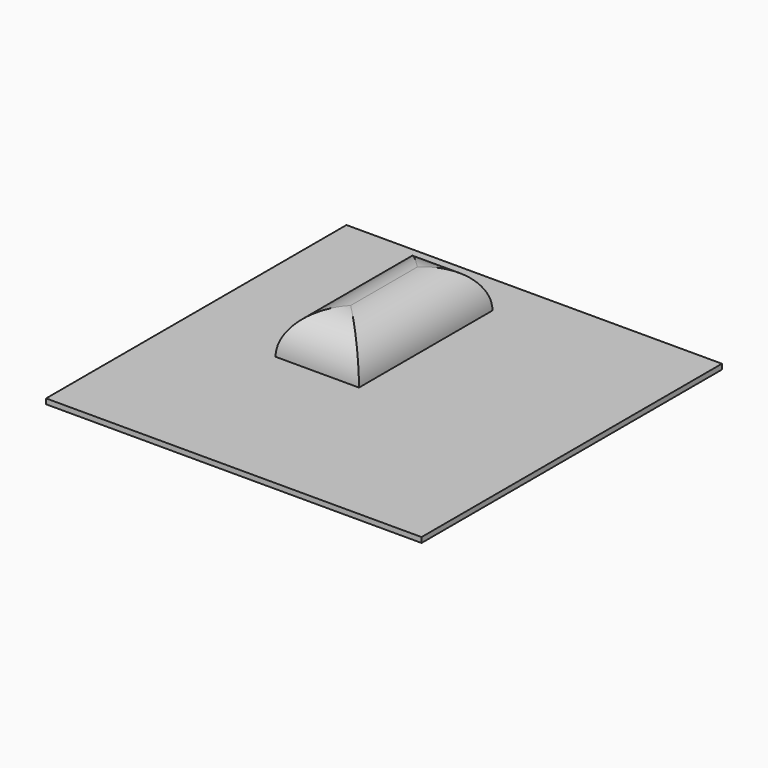
from build123d import *

# Parameters (mm, degrees)
F0_W     = 50.8
F0_H     = 101.6
F1_DEPTH = 25.4
F2_R     = 25.39999
F4_W     = 228.6
F4_H     = 228.6
F5_DEPTH = 3.175


# Not quite as in the source:
# - a fillet or chamfer is up to 0.001 mm smaller than in the source, because OpenCascade refuses the exact size


with BuildPart() as f1:
    # F0 (on Top) → F1 (new body)
    with BuildSketch(Plane.XY):
        Rectangle(F0_W, F0_H)
    extrude(amount=F1_DEPTH)

    # F2 (radius 25.4 in the source; OpenCascade refuses exactly that, so slightly less here)
    f2_edges = [f1.edges().sort_by_distance(p)[0] for p in [
        (-25.4, 0, 25.4),
        (0, -50.8, 25.4),
        (25.4, 0, 25.4),
        (0, 50.8, 25.4),
    ]]
    fillet(f2_edges, radius=F2_R)


with BuildPart() as f5:
    # F4 (on offset) → F5 (new body)
    with BuildSketch(Plane.XY.offset(-25.4)):
        Rectangle(F4_W, F4_H)
    extrude(amount=-F5_DEPTH)


solid = Compound([f1.part, f5.part])
